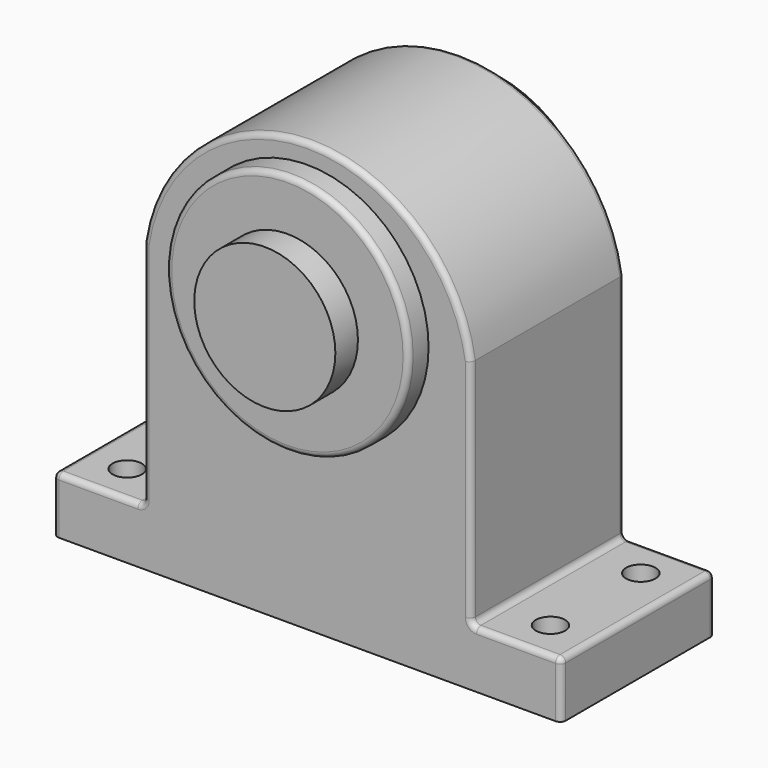
from build123d import *

# Parameters (mm, degrees)
F1_DEPTH       = 170
F2_R           = 107.5
F3_DEPTH       = 22
F4_R           = 107.5
F5_DEPTH       = 22
F6_R           = 13
F7_DEPTH       = 380.001
F8_T1_DEPTH    = 170
F8_T3_DEPTH    = 57.5
F8_T5_DEPTH    = 160
F8_T7_DEPTH    = 237.5
F8_T9_DEPTH    = 70
F8_T11_DEPTH   = 70
F8_S15_W       = 5.1
F8_S15_H       = 5.1
F8_T16_DEPTH   = 5.1
F8_S21_W       = 5.1
F8_S21_H       = 5.1
F8_T22_DEPTH   = 5.1
F8_S27_W       = 5.1
F8_S27_H       = 5.1
F8_T28_DEPTH   = 5.1
F8_S33_W       = 5.1
F8_S33_H       = 5.1
F8_T34_DEPTH   = 5.1
F8_T38_ANGLE   = 172.8380794601
F8_T40_ANGLE   = 172.8380794601
F8_T44_ANGLE   = 90
F8_T46_ANGLE   = 90
F8_T48_ANGLE   = 90
F8_T50_ANGLE   = 90
F9_R           = 62.5
F10_DEPTH      = 240
F10_DEPTH_BACK = 25


# Not quite as in the source:
# - a fillet or chamfer that OpenCascade refuses, or shapes differently, is made with other operations: its cross-section is extruded or revolved along the edge and cut away or added


with BuildPart() as f1:
    # F0 (on Front) → F1 (new body)
    with BuildSketch(Plane.XZ):
        with BuildLine():
            Line((145, 0), (90, 0))
            ThreePointArc((90, 0), (63.6396103068, -63.6396103068), (0, -90))
            Line((0, -90), (0, -255))
            Line((0, -255), (225, -255))
            Line((225, -255), (225, -205))
            Line((225, -205), (145, -205))
            Line((145, -205), (145, 0))
        make_face()
        with BuildLine():
            ThreePointArc((-90, 0), (0, 90), (90, 0))
            Line((90, 0), (145, 0))
            ThreePointArc((145, 0), (0, 125), (-145, 0))
            Line((-145, 0), (-90, 0))
        make_face()
        with BuildLine():
            ThreePointArc((-55, 0), (0, 55), (55, 0))
            Line((55, 0), (90, 0))
            ThreePointArc((90, 0), (0, 90), (-90, 0))
            Line((-90, 0), (-55, 0))
        make_face()
        with BuildLine():
            ThreePointArc((0, -90), (-63.6396103068, -63.6396103068), (-90, 0))
            Line((-90, 0), (-145, 0))
            Line((-145, 0), (-145, -205))
            Line((-145, -205), (-225, -205))
            Line((-225, -205), (-225, -255))
            Line((-225, -255), (0, -255))
            Line((0, -255), (0, -90))
        make_face()
        with BuildLine():
            ThreePointArc((0, -55), (-38.8908729653, -38.8908729653), (-55, 0))
            Line((-55, 0), (-90, 0))
            ThreePointArc((-90, 0), (-63.6396103068, -63.6396103068), (0, -90))
            Line((0, -90), (0, -55))
        make_face()
        with BuildLine():
            Line((90, 0), (55, 0))
            ThreePointArc((55, 0), (38.8908729653, -38.8908729653), (0, -55))
            Line((0, -55), (0, -90))
            ThreePointArc((0, -90), (63.6396103068, -63.6396103068), (90, 0))
        make_face()
        with BuildLine():
            ThreePointArc((0, -55), (38.8908729653, -38.8908729653), (55, 0))
            Line((55, 0), (0, 0))
            Line((0, 0), (0, -55))
        make_face()
        with BuildLine():
            Line((0, 0), (-55, 0))
            ThreePointArc((-55, 0), (-38.8908729653, -38.8908729653), (0, -55))
            Line((0, -55), (0, 0))
        make_face()
        with BuildLine():
            Line((0, 0), (55, 0))
            ThreePointArc((55, 0), (0, 55), (-55, 0))
            Line((-55, 0), (0, 0))
        make_face()
    extrude(amount=F1_DEPTH)

    # F4 (on face) → F5 (join)
    with BuildSketch(Plane.XZ.offset(170)):
        Circle(F4_R)
    extrude(amount=F5_DEPTH)

    # F6 (on face) → F7 (cut, through all)
    with BuildSketch(Plane(origin=(0, 0, -255), x_dir=(1, 0, 0), z_dir=(0, 0, -1))):
        with Locations((-187.5, 135)):
            Circle(F6_R)
        with Locations((-187.5, 35)):
            Circle(F6_R)
        with Locations((187.5, 135)):
            Circle(F6_R)
        with Locations((187.5, 35)):
            Circle(F6_R)
    extrude(amount=-F7_DEPTH, mode=Mode.SUBTRACT)

    # F8: fillet of radius 5 on 19 edges, made by hand

    # F8_s2 → F8_t1 (join)
    with BuildSketch(Plane.XZ):
        with BuildLine():
            ThreePointArc((150, -205), (146.4644660941, -203.5355339059), (145, -200))
            Line((145, -200), (145, -205))
            Line((145, -205), (150, -205))
        make_face()
        with BuildLine():
            ThreePointArc((-145, -200), (-146.4644660941, -203.5355339059), (-150, -205))
            Line((-150, -205), (-145, -205))
            Line((-145, -205), (-145, -200))
        make_face()
    extrude(amount=F8_T1_DEPTH)

    # F8_s4 → F8_t3 (cut)
    with BuildSketch(Plane.XY.offset(-267.5)):
        with BuildLine():
            ThreePointArc((-220, 0), (-223.5355339059, -1.4644660941), (-225, -5))
            Line((-225, -5), (-225, 0))
            Line((-225, 0), (-220, 0))
        make_face()
        with BuildLine():
            ThreePointArc((-220, -170), (-223.5355339059, -168.5355339059), (-225, -165))
            Line((-225, -165), (-225, -170))
            Line((-225, -170), (-220, -170))
        make_face()
        with BuildLine():
            ThreePointArc((225, -5), (223.5355339059, -1.4644660941), (220, 0))
            Line((220, 0), (225, 0))
            Line((225, 0), (225, -5))
        make_face()
        with BuildLine():
            ThreePointArc((225, -165), (223.5355339059, -168.5355339059), (220, -170))
            Line((220, -170), (225, -170))
            Line((225, -170), (225, -165))
        make_face()
    extrude(amount=F8_T3_DEPTH, mode=Mode.SUBTRACT)

    # F8_s6 → F8_t5 (cut)
    with BuildSketch(Plane.XZ.offset(5)):
        with BuildLine():
            ThreePointArc((-225, -210), (-223.5355339059, -206.4644660941), (-220, -205))
            Line((-220, -205), (-225, -205))
            Line((-225, -205), (-225, -210))
        make_face()
        with BuildLine():
            ThreePointArc((225, -210), (223.5355339059, -206.4644660941), (220, -205))
            Line((220, -205), (225, -205))
            Line((225, -205), (225, -210))
        make_face()
    extrude(amount=F8_T5_DEPTH, mode=Mode.SUBTRACT)

    # F8_s8 → F8_t7 (cut)
    with BuildSketch(Plane.XY.offset(-200)):
        with BuildLine():
            ThreePointArc((-140, 0), (-143.5355339059, -1.4644660941), (-145, -5))
            Line((-145, -5), (-145, 0))
            Line((-145, 0), (-140, 0))
        make_face()
        with BuildLine():
            ThreePointArc((-140, -170), (-143.5355339059, -168.5355339059), (-145, -165))
            Line((-145, -165), (-145, -170))
            Line((-145, -170), (-140, -170))
        make_face()
        with BuildLine():
            ThreePointArc((140, 0), (143.5355339059, -1.4644660941), (145, -5))
            Line((145, -5), (145, 0))
            Line((145, 0), (140, 0))
        make_face()
        with BuildLine():
            ThreePointArc((140, -170), (143.5355339059, -168.5355339059), (145, -165))
            Line((145, -165), (145, -170))
            Line((145, -170), (140, -170))
        make_face()
    extrude(amount=F8_T7_DEPTH, mode=Mode.SUBTRACT)

    # F8_s10 → F8_t9 (cut)
    with BuildSketch(Plane.YZ.offset(-220)):
        with BuildLine():
            ThreePointArc((0, -210), (-1.4644660941, -206.4644660941), (-5, -205))
            Line((-5, -205), (0, -205))
            Line((0, -205), (0, -210))
        make_face()
        with BuildLine():
            ThreePointArc((-170, -210), (-168.5355339059, -206.4644660941), (-165, -205))
            Line((-165, -205), (-170, -205))
            Line((-170, -205), (-170, -210))
        make_face()
    extrude(amount=F8_T9_DEPTH, mode=Mode.SUBTRACT)

    # F8_s12 → F8_t11 (cut)
    with BuildSketch(Plane.YZ.offset(150)):
        with BuildLine():
            ThreePointArc((-5, -205), (-1.4644660941, -206.4644660941), (0, -210))
            Line((0, -210), (0, -205))
            Line((0, -205), (-5, -205))
        make_face()
        with BuildLine():
            ThreePointArc((-165, -205), (-168.5355339059, -206.4644660941), (-170, -210))
            Line((-170, -210), (-170, -205))
            Line((-170, -205), (-165, -205))
        make_face()
    extrude(amount=F8_T11_DEPTH, mode=Mode.SUBTRACT)


with BuildPart() as f3:
    # F2 (on face) → F3 (new body)
    with BuildSketch(Plane(origin=(0, 0, 0), x_dir=(-1, 0, 0), z_dir=(0, 1, 0))):
        Circle(F2_R)
    extrude(amount=F3_DEPTH)

    # F8#2: fillet of radius 5 on 1 edges, made by hand

    # F8_2_s1 → F8_2_t2 (revolve, cut)
    with BuildSketch(Plane.XY):
        with BuildLine():
            ThreePointArc((-107.5, 17), (-106.0355339059, 20.5355339059), (-102.5, 22))
            Line((-102.5, 22), (-107.5, 22))
            Line((-107.5, 22), (-107.5, 17))
        make_face()
    revolve(axis=Axis((0, 22, 0), (0, 1, 0)), mode=Mode.SUBTRACT)


with BuildPart() as f8_tool14:
    # F8_s15 → F8_t16 (new body)
    with BuildSketch(Plane.XZ.offset(5)):
        with Locations((-222.55, -207.45)):
            Rectangle(F8_S15_W, F8_S15_H)
    extrude(amount=-F8_T16_DEPTH)

    # F8_s17 → F8_t18 (revolve, cut)
    with BuildSketch(Plane(origin=(-220, -5, -210), x_dir=(0.7071067812, 0, -0.7071067812), z_dir=(0.7071067812, 0, 0.7071067812))):
        with BuildLine():
            ThreePointArc((0, -5), (5, 0), (0, 5))
            Line((0, 5), (0, -5))
        make_face()
    revolve(axis=Axis((-220, -5, -210), (0, 1, 0)), mode=Mode.SUBTRACT)


with BuildPart() as f1_1:
    add(f1.part)

    # F8_t13: cut F8_tool14
    add(f8_tool14.part, mode=Mode.SUBTRACT)


with BuildPart() as f8_tool20:
    # F8_s21 → F8_t22 (new body)
    with BuildSketch(Plane.XZ.offset(165)):
        with Locations((-222.55, -207.45)):
            Rectangle(F8_S21_W, F8_S21_H)
    extrude(amount=F8_T22_DEPTH)

    # F8_s23 → F8_t24 (revolve, cut)
    with BuildSketch(Plane(origin=(-220, -165, -210), x_dir=(0.7071067812, 0, -0.7071067812), z_dir=(-0.7071067812, 0, -0.7071067812))):
        with BuildLine():
            ThreePointArc((0, -5), (5, 0), (0, 5))
            Line((0, 5), (0, -5))
        make_face()
    revolve(axis=Axis((-220, -165, -210), (0, -1, 0)), mode=Mode.SUBTRACT)


with BuildPart() as f1_2:
    add(f1_1.part)

    # F8_t19: cut F8_tool20
    add(f8_tool20.part, mode=Mode.SUBTRACT)


with BuildPart() as f8_tool26:
    # F8_s27 → F8_t28 (new body)
    with BuildSketch(Plane.YZ.offset(220)):
        with Locations((-2.45, -207.45)):
            Rectangle(F8_S27_W, F8_S27_H)
    extrude(amount=F8_T28_DEPTH)

    # F8_s29 → F8_t30 (revolve, cut)
    with BuildSketch(Plane(origin=(220, -5, -210), x_dir=(0, -0.7071067812, -0.7071067812), z_dir=(0, -0.7071067812, 0.7071067812))):
        with BuildLine():
            ThreePointArc((0, -5), (5, 0), (0, 5))
            Line((0, 5), (0, -5))
        make_face()
    revolve(axis=Axis((220, -5, -210), (1, 0, 0)), mode=Mode.SUBTRACT)


with BuildPart() as f1_3:
    add(f1_2.part)

    # F8_t25: cut F8_tool26
    add(f8_tool26.part, mode=Mode.SUBTRACT)


with BuildPart() as f8_tool32:
    # F8_s33 → F8_t34 (new body)
    with BuildSketch(Plane.YZ.offset(220)):
        with Locations((-167.55, -207.45)):
            Rectangle(F8_S33_W, F8_S33_H)
    extrude(amount=F8_T34_DEPTH)

    # F8_s35 → F8_t36 (revolve, cut)
    with BuildSketch(Plane(origin=(220, -165, -210), x_dir=(0, 0.7071067812, -0.7071067812), z_dir=(0, -0.7071067812, -0.7071067812))):
        with BuildLine():
            ThreePointArc((0, -5), (5, 0), (0, 5))
            Line((0, 5), (0, -5))
        make_face()
    revolve(axis=Axis((220, -165, -210), (1, 0, 0)), mode=Mode.SUBTRACT)


with BuildPart() as f1_4:
    add(f1_3.part)

    # F8_t31: cut F8_tool32
    add(f8_tool32.part, mode=Mode.SUBTRACT)

    # F8_s37 → F8_t38 (revolve, cut)
    with BuildSketch(Plane(origin=(1.3464774141, 0, -21.5157360257), x_dir=(0, 1, 0), z_dir=(0.0624588658, 0, -0.998047539))):
        with BuildLine():
            ThreePointArc((0, 140.2508884983), (-1.4644660941, 143.7864224042), (-5, 145.2508884983))
            Line((-5, 145.2508884983), (0, 145.2508884983))
            Line((0, 145.2508884983), (0, 140.2508884983))
        make_face()
    revolve(axis=Axis((0, 0, -21.6), (0, -1, 0)), revolution_arc=F8_T38_ANGLE, mode=Mode.SUBTRACT)

    # F8_s39 → F8_t40 (revolve, cut)
    with BuildSketch(Plane(origin=(1.3464774141, 0, -21.5157360257), x_dir=(0, 1, 0), z_dir=(0.0624588658, 0, -0.998047539))):
        with BuildLine():
            ThreePointArc((-170, 140.2508884983), (-168.5355339059, 143.7864224042), (-165, 145.2508884983))
            Line((-165, 145.2508884983), (-170, 145.2508884983))
            Line((-170, 145.2508884983), (-170, 140.2508884983))
        make_face()
    revolve(axis=Axis((0, -170, -21.6), (0, -1, 0)), revolution_arc=F8_T40_ANGLE, mode=Mode.SUBTRACT)

    # F8_s41 → F8_t42 (revolve, cut)
    with BuildSketch(Plane.XY):
        with BuildLine():
            ThreePointArc((107.5, -187), (106.0355339059, -190.5355339059), (102.5, -192))
            Line((102.5, -192), (107.5, -192))
            Line((107.5, -192), (107.5, -187))
        make_face()
    revolve(axis=Axis((0, -192, 0), (0, -1, 0)), mode=Mode.SUBTRACT)

    # F8_s43 → F8_t44 (revolve, cut)
    with BuildSketch(Plane.YZ.offset(150)):
        with BuildLine():
            ThreePointArc((-170, -210), (-168.5355339059, -206.4644660941), (-165, -205))
            Line((-165, -205), (-170, -205))
            Line((-170, -205), (-170, -210))
        make_face()
    revolve(axis=Axis((150, -170, -200), (0, 1, 0)), revolution_arc=F8_T44_ANGLE, mode=Mode.SUBTRACT)

    # F8_s45 → F8_t46 (revolve, cut)
    with BuildSketch(Plane.YZ.offset(150)):
        with BuildLine():
            ThreePointArc((0, -210), (-1.4644660941, -206.4644660941), (-5, -205))
            Line((-5, -205), (0, -205))
            Line((0, -205), (0, -210))
        make_face()
    revolve(axis=Axis((150, 0, -200), (0, 1, 0)), revolution_arc=F8_T46_ANGLE, mode=Mode.SUBTRACT)

    # F8_s47 → F8_t48 (revolve, cut)
    with BuildSketch(Plane.XY.offset(-200)):
        with BuildLine():
            ThreePointArc((-140, -170), (-143.5355339059, -168.5355339059), (-145, -165))
            Line((-145, -165), (-145, -170))
            Line((-145, -170), (-140, -170))
        make_face()
    revolve(axis=Axis((-150, -170, -200), (0, 1, 0)), revolution_arc=F8_T48_ANGLE, mode=Mode.SUBTRACT)

    # F8_s49 → F8_t50 (revolve, cut)
    with BuildSketch(Plane.XY.offset(-200)):
        with BuildLine():
            ThreePointArc((-140, 0), (-143.5355339059, -1.4644660941), (-145, -5))
            Line((-145, -5), (-145, 0))
            Line((-145, 0), (-140, 0))
        make_face()
    revolve(axis=Axis((-150, 0, -200), (0, 1, 0)), revolution_arc=F8_T50_ANGLE, mode=Mode.SUBTRACT)


with BuildPart() as f10:
    # F9 (on face) → F10 (new body, two sides)
    with BuildSketch(Plane.XZ.offset(192)) as f10_sk:
        Circle(F9_R)
    extrude(amount=-F10_DEPTH)
    extrude(f10_sk.sketch, amount=F10_DEPTH_BACK)


solid = Compound([f3.part, f1_4.part, f10.part])
